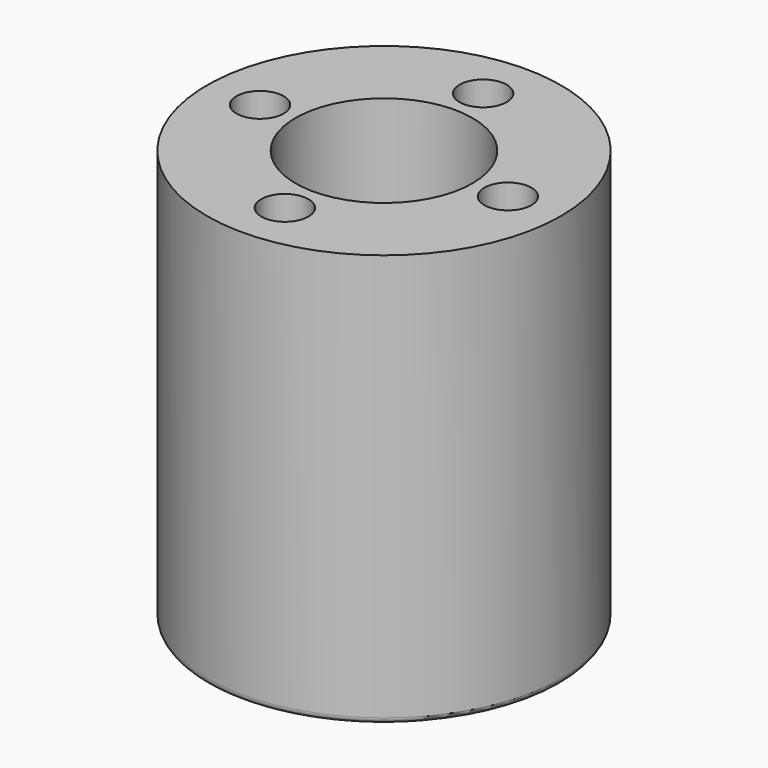
from build123d import *

# Parameters (mm, degrees)
F0_R     = 30
F0_R_2   = 4
F0_R_3   = 15
F1_DEPTH = 70
F2_R     = 1.99999
F3_R     = 1


# Not quite as in the source:
# - a fillet or chamfer is up to 0.001 mm smaller than in the source, because OpenCascade refuses the exact size


with BuildPart() as f1:
    # F0 (on Top) → F1 (new body)
    with BuildSketch(Plane.XY):
        Circle(F0_R)
        with Locations((0, -21)):
            Circle(F0_R_2, mode=Mode.SUBTRACT)
        with Locations((-21, 0)):
            Circle(F0_R_2, mode=Mode.SUBTRACT)
        Circle(F0_R_3, mode=Mode.SUBTRACT)
        with Locations((21, 0)):
            Circle(F0_R_2, mode=Mode.SUBTRACT)
        with Locations((0, 21)):
            Circle(F0_R_2, mode=Mode.SUBTRACT)
    extrude(amount=F1_DEPTH)

    # F2 (radius 2 in the source; OpenCascade refuses exactly that, so slightly less here)
    f2_edges = [f1.edges().sort_by_distance(p)[0] for p in [
        (-15, 0, 0),
    ]]
    fillet(f2_edges, radius=F2_R)

    # F3
    f3_edges = [f1.edges().sort_by_distance(p)[0] for p in [
        (-30, 0, 0),
    ]]
    fillet(f3_edges, radius=F3_R)


solid = f1.part
